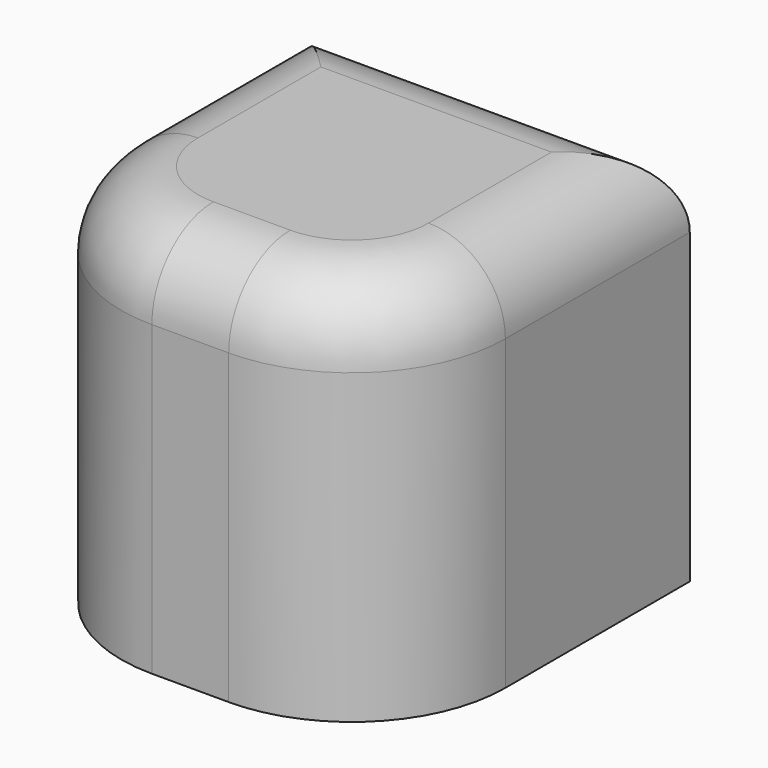
from build123d import *

# Parameters (mm, degrees)
F0_W        = 25
F0_H        = 25
F1_DEPTH    = 25
F2_R        = 5
F3_T1_DEPTH = 25
F3_T4_ANGLE = 90
F3_T6_ANGLE = 90


# Not quite as in the source:
# - a fillet or chamfer that OpenCascade refuses, or shapes differently, is made with other operations: its cross-section is extruded or revolved along the edge and cut away or added


with BuildPart() as f1:
    # F0 (on Top) → F1 (new body)
    with BuildSketch(Plane.XY):
        Rectangle(F0_W, F0_H)
    extrude(amount=F1_DEPTH)

    # F2
    f2_edges = [f1.edges().sort_by_distance(p)[0] for p in [
        (0, 12.5, 25),
        (-12.5, 0, 25),
        (0, -12.5, 25),
        (12.5, 0, 25),
    ]]
    fillet(f2_edges, radius=F2_R)

    # F3: fillet of radius 10 on 2 edges, made by hand

    # F3_s2 → F3_t1 (cut)
    with BuildSketch(Plane.XY):
        with BuildLine():
            ThreePointArc((12.5, -2.5), (9.5710678119, -9.5710678119), (2.5, -12.5))
            Line((2.5, -12.5), (2.5, -12.7))
            Line((2.5, -12.7), (12.7, -12.7))
            Line((12.7, -12.7), (12.7, -2.5))
            Line((12.7, -2.5), (12.5, -2.5))
        make_face()
        with BuildLine():
            ThreePointArc((-12.5, -2.5), (-9.5710678119, -9.5710678119), (-2.5, -12.5))
            Line((-2.5, -12.5), (-2.5, -12.7))
            Line((-2.5, -12.7), (-12.7, -12.7))
            Line((-12.7, -12.7), (-12.7, -2.5))
            Line((-12.7, -2.5), (-12.5, -2.5))
        make_face()
    extrude(amount=F3_T1_DEPTH, mode=Mode.SUBTRACT)

    # F3_s3 → F3_t4 (revolve, cut)
    with BuildSketch(Plane.XZ.offset(2.5)):
        with BuildLine():
            ThreePointArc((-7.5, 25), (-11.0355339059, 23.5355339059), (-12.5, 20))
            Line((-12.5, 20), (-12.5, 25))
            Line((-12.5, 25), (-7.5, 25))
        make_face()
    revolve(axis=Axis((-2.5, -2.5, 25), (0, 0, 1)), revolution_arc=F3_T4_ANGLE, mode=Mode.SUBTRACT)

    # F3_s5 → F3_t6 (revolve, cut)
    with BuildSketch(Plane.YZ.offset(2.5)):
        with BuildLine():
            ThreePointArc((-7.5, 25), (-11.0355339059, 23.5355339059), (-12.5, 20))
            Line((-12.5, 20), (-12.5, 25))
            Line((-12.5, 25), (-7.5, 25))
        make_face()
    revolve(axis=Axis((2.5, -2.5, 25), (0, 0, 1)), revolution_arc=F3_T6_ANGLE, mode=Mode.SUBTRACT)


solid = f1.part
